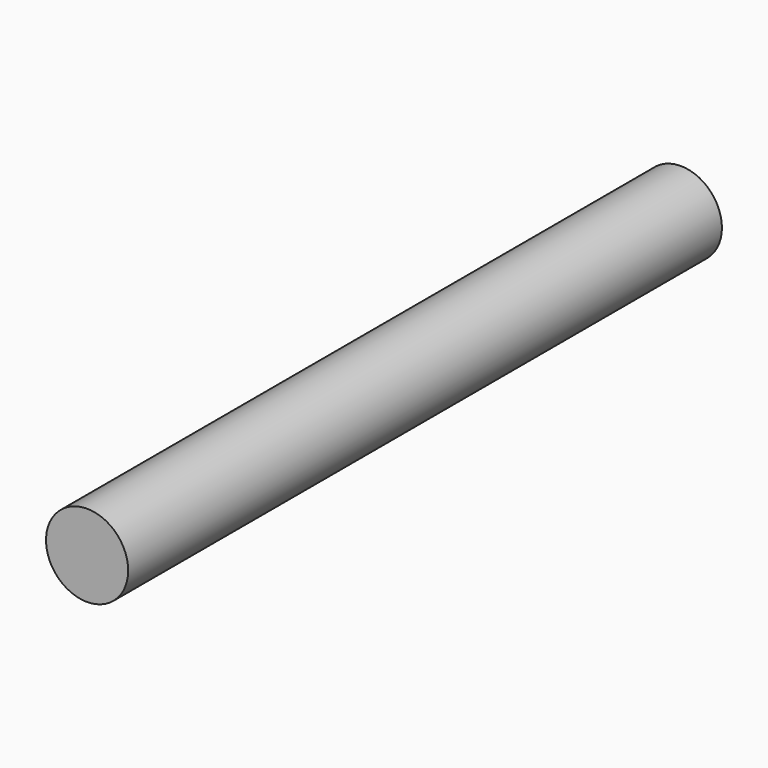
from build123d import *

# Parameters (mm, degrees)
F0_R     = 12.5
F1_DEPTH = 225.806


# Not quite as in the source:
# - the program builds the solid bodies; features that only make, move or delete a surface that nothing else refers to are left out


with BuildPart() as f1:
    # F0 (on Front) → F1 (new body)
    with BuildSketch(Plane.XZ):
        with Locations((-125.2229064703, 56.0913495719)):
            Circle(F0_R)
    extrude(amount=F1_DEPTH)


solid = f1.part
